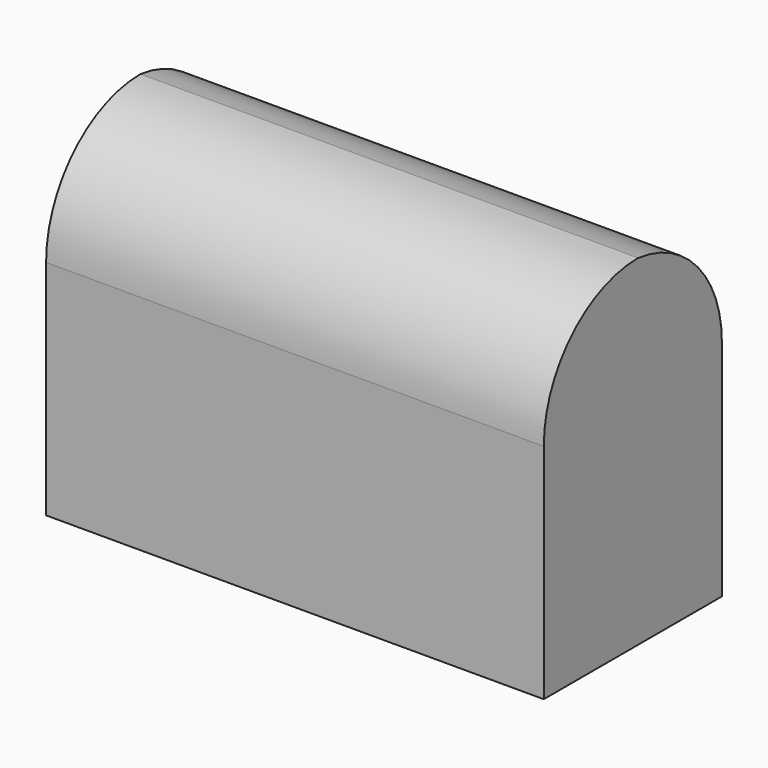
from build123d import *

# Parameters (mm, degrees)
F0_W        = 38
F0_H        = 26
F1_DEPTH    = 17
F2_R        = 9
F3_T1_DEPTH = 82.72135955


# Not quite as in the source:
# - a fillet or chamfer that OpenCascade refuses, or shapes differently, is made with other operations: its cross-section is extruded or revolved along the edge and cut away or added


with BuildPart() as f1:
    # F0 (on Front) → F1 (new body)
    with BuildSketch(Plane.XZ):
        with Locations((19, 13)):
            Rectangle(F0_W, F0_H)
    extrude(amount=F1_DEPTH)

    # F2
    f2_edges = [f1.edges().sort_by_distance(p)[0] for p in [
        (19, -17, 26),
    ]]
    fillet(f2_edges, radius=F2_R)

    # F3: fillet of radius 9 on 1 edges, made by hand

    # F3_s2 → F3_t1 (cut)
    with BuildSketch(Plane.YZ.offset(-22.360679775)):
        with BuildLine():
            ThreePointArc((-8, 26), (-2.2917960675, 23.05572809), (0, 17.05572809))
            Line((0, 17.05572809), (0, 26))
            Line((0, 26), (-8, 26))
        make_face()
    extrude(amount=F3_T1_DEPTH, mode=Mode.SUBTRACT)


solid = f1.part
